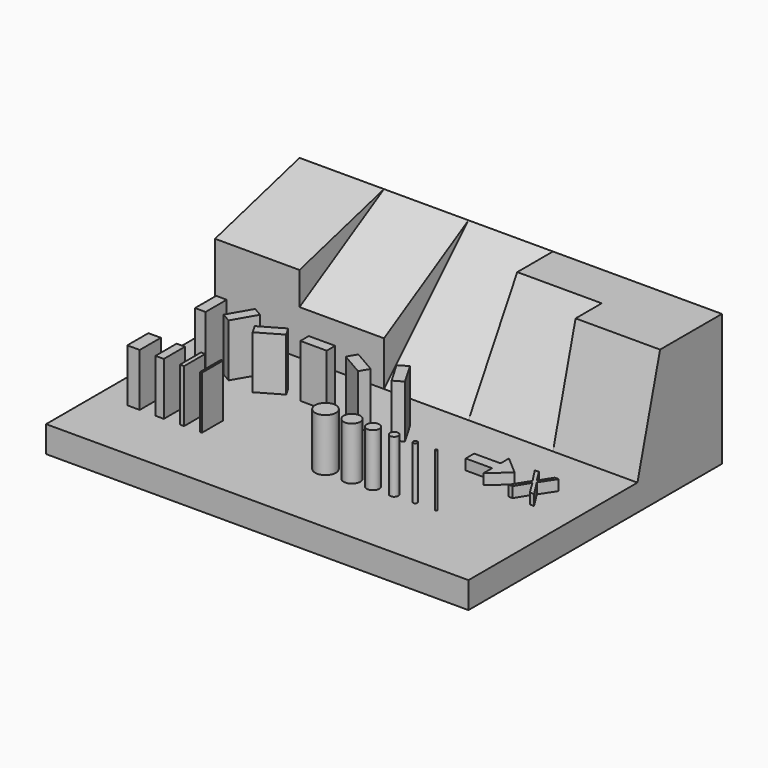
from build123d import *

# Parameters (mm, degrees)
F0_W          = 101.6
F0_H          = 76.2
F1_DEPTH      = 6.35
F2_W          = 101.6
F2_H          = 25.4
F3_DEPTH      = 25.4
F5_DEPTH      = 20.32
F7_DEPTH      = 20.32
F9_DEPTH      = 20.32
F11_DEPTH     = 20.32
F13_DEPTH     = 25.4
F15_W         = 2.54
F15_H         = 6.35
F15_W_2       = 6.35
F15_H_2       = 2.54
F16_DEPTH     = 12.7
F17_W         = 3
F17_H         = 6.35
F17_W_2       = 2
F17_W_3       = 1
F18_DEPTH     = 12.7
F19_R         = 1.5
F19_R_2       = 1
F19_R_3       = 0.25
F19_R_4       = 0.5
F19_W         = 0.5
F19_H         = 6.35
F19_R_5       = 2
F19_R_6       = 2.5
F20_DEPTH     = 12.7
F21_W         = 6.35
F21_H         = 2.54
F21_TEXT_SIZE = 10.7357912283
F22_DEPTH     = 2.54
F14_TEXT_SIZE = 5.7168951672
F23_DEPTH     = 2.54


# Not quite as in the source:
# - Text() gives the source's letters only with a copy of the font that has no kerning and outlines rounded to 1/6400 em; it was checked with that copy


with BuildPart() as f1:
    # F0 (on Top) → F1 (new body)
    with BuildSketch(Plane.XY):
        with Locations((1.2065004557, 9.7788204194)):
            Rectangle(F0_W, F0_H)
    extrude(amount=F1_DEPTH)

    # F2 (on face) → F3 (join)
    with BuildSketch(Plane.XY.offset(6.35)):
        with Locations((1.2065004557, 35.1788204194)):
            Rectangle(F2_W, F2_H)
    extrude(amount=F3_DEPTH)

    # F4 (on face) → F5 (cut)
    with BuildSketch(Plane(origin=(-49.5934995443, 0, 0), x_dir=(0, -1, 0), z_dir=(-1, 0, 0))):
        Polygon((-22.4788204194, 31.75), (-47.8788204194, 31.75), (-22.4788204194, 24.9440905122), align=None)
    extrude(amount=-F5_DEPTH, mode=Mode.SUBTRACT)

    # F6 (on face) → F7 (cut)
    with BuildSketch(Plane(origin=(-29.2734995443, 0, 0), x_dir=(0, -1, 0), z_dir=(-1, 0, 0))):
        Polygon((-22.4788204194, 31.75), (-47.8788204194, 31.75), (-22.4788204194, 17.0853031626), align=None)
    extrude(amount=-F7_DEPTH, mode=Mode.SUBTRACT)

    # F8 (on face) → F9 (cut)
    with BuildSketch(Plane(origin=(-8.9534995443, 0, 0), x_dir=(0, -1, 0), z_dir=(-1, 0, 0))):
        Polygon((-22.4788204194, 31.75), (-47.8788204194, 31.75), (-22.4788204194, 6.35), align=None)
    extrude(amount=-F9_DEPTH, mode=Mode.SUBTRACT)

    # F10 (on face) → F11 (cut)
    with BuildSketch(Plane(origin=(11.3665004557, 0, 0), x_dir=(0, -1, 0), z_dir=(-1, 0, 0))):
        Polygon((-22.4788204194, 6.35), (-22.4788204194, 31.75), (-37.1435172568, 31.75), align=None)
    extrude(amount=-F11_DEPTH, mode=Mode.SUBTRACT)

    # F12 (on face) → F13 (cut)
    with BuildSketch(Plane(origin=(31.6865004557, 0, 0), x_dir=(0, -1, 0), z_dir=(-1, 0, 0))):
        Polygon((-22.4788204194, 6.35), (-22.4788204194, 31.75), (-29.2847299072, 31.75), align=None)
    extrude(amount=-F13_DEPTH, mode=Mode.SUBTRACT)

    # F15 (on face) → F16 (join)
    with BuildSketch(Plane.XY.offset(6.35)):
        Polygon((-30.7567966722, 12.4730551788), (-32.9565011978, 13.7430551788), (-36.1315011978, 8.2437938648), (-33.9317966722, 6.9737938648), align=None)
        with Locations((-40.7336540531, 10.1487938648)):
            Rectangle(F15_W, F15_H)
        Polygon((-21.8797739216, 9.2190893392), (-23.1497739216, 11.4187938648), (-28.6490352356, 8.2437938648), (-27.3790352356, 6.0440893392), align=None)
        with Locations((-15.0200079698, 10.1487938648)):
            Rectangle(F15_W_2, F15_H_2)
        Polygon((-2.0435631671, 6.0440893392), (-0.7735631671, 8.2437938648), (-6.2728244811, 11.4187938648), (-7.5428244811, 9.2190893392), align=None)
        Polygon((5.2540015559, 6.9737938648), (7.4537060816, 8.2437938648), (4.2787060816, 13.7430551788), (2.0790015559, 12.4730551788), align=None)
    extrude(amount=F16_DEPTH)

    # F17 (on face) → F18 (join)
    with BuildSketch(Plane.XY.offset(6.35)):
        with Locations((-40.9636540531, -9.6536359814)):
            Rectangle(F17_W, F17_H)
        with Locations((-34.6536540531, -9.6656826407)):
            Rectangle(F17_W_2, F17_H)
        with Locations((-29.3436540531, -9.6072374925)):
            Rectangle(F17_W_3, F17_H)
    extrude(amount=F18_DEPTH)

    # F19 (on face) → F20 (join)
    with BuildSketch(Plane.XY.offset(6.35)):
        with Locations((14.2211687403, -9.78958701)):
            Circle(F19_R)
        with Locations((19.3011687403, -9.78958701)):
            Circle(F19_R_2)
        with Locations((29.4611687403, -9.78958701)):
            Circle(F19_R_3)
        with Locations((24.3811687403, -9.78958701)):
            Circle(F19_R_4)
        with Locations((-24.7836540531, -9.6072374925)):
            Rectangle(F19_W, F19_H)
        with Locations((9.1411687403, -9.78958701)):
            Circle(F19_R_5)
        with Locations((2.7911687403, -9.78958701)):
            Circle(F19_R_6)
    extrude(amount=F20_DEPTH)

    # F21 (on face) → F22 (join)
    with BuildSketch(Plane.XY.offset(6.35)):
        with Locations((26.8964441493, 7.4653104874)):
            Rectangle(F21_W, F21_H)
        Polygon((30.0714441493, 11.2753104874), (30.0714441493, 8.7353104874), (30.0714441493, 6.1953104874), (30.0714441493, 3.6553104874), (34.4629101455, 7.4653104874), align=None)
        with Locations((36.6403087974, 2.8932206333)):
            Text('X', F21_TEXT_SIZE, font='Open Sans', text_align=(TextAlign.LEFT, TextAlign.BOTTOM))
    extrude(amount=F22_DEPTH)

    # F14 (on face) → F23 (cut)
    with BuildSketch(Plane(origin=(0, 47.8788204194, 0), x_dir=(-1, 0, 0), z_dir=(0, 1, 0))):
        with Locations((-47.9095391929, 19.1273186356)):
            Text('75°', F14_TEXT_SIZE, font='Open Sans', text_align=(TextAlign.LEFT, TextAlign.BOTTOM))
        with Locations((-25.4971999675, 16.6211063042)):
            Text('60°', F14_TEXT_SIZE, font='Open Sans', text_align=(TextAlign.LEFT, TextAlign.BOTTOM))
        with Locations((-4.8813298345, 19.1273186356)):
            Text('45°', F14_TEXT_SIZE, font='Open Sans', text_align=(TextAlign.LEFT, TextAlign.BOTTOM))
        with Locations((16.0371419042, 20.7372708246)):
            Text('30°', F14_TEXT_SIZE, font='Open Sans', text_align=(TextAlign.LEFT, TextAlign.BOTTOM))
        with Locations((30.4985493422, 15.875)):
            Text('15°', F14_TEXT_SIZE, font='Open Sans', text_align=(TextAlign.LEFT, TextAlign.BOTTOM))
    extrude(amount=-F23_DEPTH, mode=Mode.SUBTRACT)


solid = f1.part
